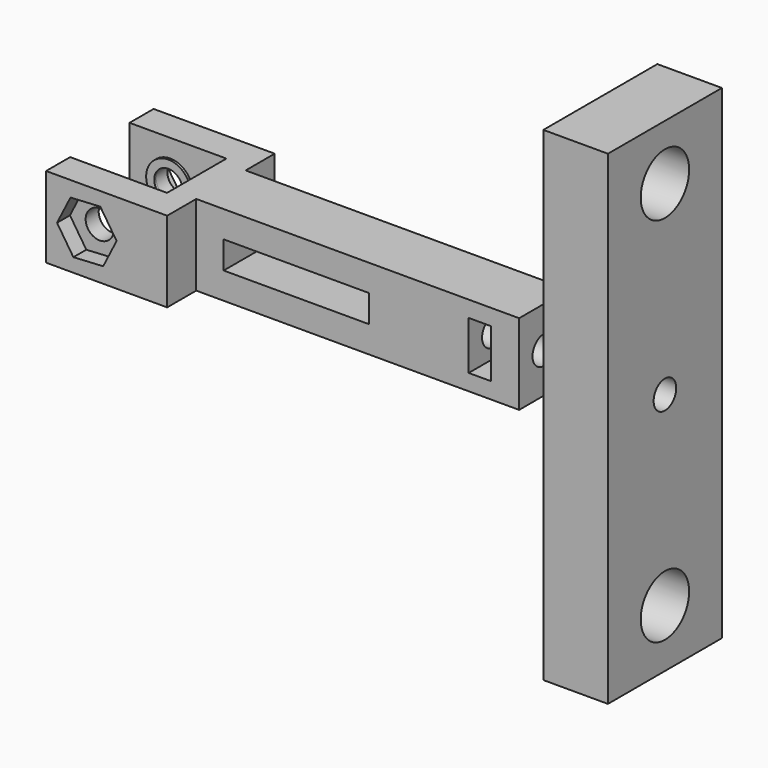
from build123d import *

# Parameters (mm, degrees)
F0_W      = 40
F0_H      = 3.825
F1_DEPTH  = 10
F2_R      = 1.75
F3_DEPTH  = 16.651
F4_W      = 18
F4_H      = 3.4
F4_W_2    = 2.75
F4_H_2    = 6
F5_DEPTH  = 12.151
F6_R      = 1.75
F7_DEPTH  = 15
F10_DEPTH = 2
F11_W     = 17.65
F11_H     = 60
F12_DEPTH = 8
F13_R     = 1.75
F14_DEPTH = 70.001
F15_R     = 2.75
F15_R_2   = 1.75
F16_DEPTH = 0.3
F17_R     = 1.75
F18_DEPTH = 2
F20_D     = 7.5


# Not quite as in the source:
# - a pattern or mirror of a feature is missing from the dataset's text; its kind, count and spacing are read off the source's solid


with BuildPart() as f1:
    # F0 (on Top) → F1 (new body)
    with BuildSketch(Plane.XY):
        Polygon((0, -3.825), (0, 0), (-3, 0), (-3, -4.6), (-15, -4.6), (-15, -8.325), (0, -8.325), align=None)
        Polygon((-3, 0), (0, 0), (0, 3.825), (0, 8.325), (-15, 8.325), (-15, 4.6), (-3, 4.6), align=None)
        with Locations((20, 1.9125)):
            Rectangle(F0_W, F0_H)
        with Locations((20, -1.9125)):
            Rectangle(F0_W, F0_H)
    extrude(amount=F1_DEPTH)

    # F2 (on face) → F3 (cut, through all)
    with BuildSketch(Plane.XZ.offset(8.325)):
        with Locations((-9.9527407438, 5)):
            Circle(F2_R)
    extrude(amount=-F3_DEPTH, mode=Mode.SUBTRACT)

    # F4 (on face) → F5 (cut, through all)
    with BuildSketch(Plane.XZ.offset(3.825)):
        with Locations((12.4002694301, 5)):
            Rectangle(F4_W, F4_H)
        with Locations((35.125, 5)):
            Rectangle(F4_W_2, F4_H_2)
    extrude(amount=-F5_DEPTH, mode=Mode.SUBTRACT)

    # F6 (on face) → F7 (cut)
    with BuildSketch(Plane.YZ.offset(40)):
        with Locations((0, 5)):
            Circle(F6_R)
    extrude(amount=-F7_DEPTH, mode=Mode.SUBTRACT)

    # F15 (on face) → F16 (join)
    with BuildSketch(Plane.XZ.offset(-4.6)):
        with Locations((-9.9527407438, 5)):
            Circle(F15_R)
        with Locations((-9.9527407438, 5)):
            Circle(F15_R_2, mode=Mode.SUBTRACT)
    f16 = extrude(amount=F16_DEPTH)

    # F16_copies: F16 across plane
    add(f16.mirror(Plane(origin=(0, 0, 0), x_dir=(0, 0, -1), z_dir=(0, -1, 0))))

    # F17 (on face) → F18 (cut)
    with BuildSketch(Plane.XZ.offset(8.325)):
        Polygon((-7.9284293953, 1.9088033227), (-6.2635302189, 5.2075067143), (-8.2878415673, 8.2987033916), (-11.9770520922, 8.0911966773), (-13.6419512686, 4.7924932857), (-11.6176399202, 1.7012966084), align=None)
        with Locations((-9.9527407438, 5)):
            Circle(F17_R, mode=Mode.SUBTRACT)
    f18 = extrude(amount=-F18_DEPTH, mode=Mode.SUBTRACT)

    # F18_copies: F18 across plane
    add(f18.mirror(Plane.ZX), mode=Mode.SUBTRACT)


with BuildPart() as f10:
    # F9 (on offset) → F10 (new body)
    with BuildSketch(Plane.YZ.offset(45)):
        Polygon((3.825, 0), (3.825, 10), (3.825, 19.8484882712), (-3.825, 19.8484882712), (-3.825, 10), (-3.825, 0), (-3.825, -10.1515117288), (3.825, -10.1515117288), align=None)
    extrude(amount=F10_DEPTH)

    # F11 (on face) → F12 (join)
    with BuildSketch(Plane.YZ.offset(47)):
        with Locations((0, 4.8484882712)):
            Rectangle(F11_W, F11_H)
    extrude(amount=F12_DEPTH)

    # F13 (on face) → F14 (cut, through all)
    with BuildSketch(Plane.YZ.offset(55)):
        with Locations((0, 5)):
            Circle(F13_R)
    extrude(amount=-F14_DEPTH, mode=Mode.SUBTRACT)

    # F20 (through all)
    with Locations(Plane(origin=(47, 0, 0), x_dir=(0, -1, 0), z_dir=(-1, 0, 0))):
        with Locations((0, -18), (0, 28)):
            Hole(F20_D / 2)


solid = Compound([f1.part, f10.part])
